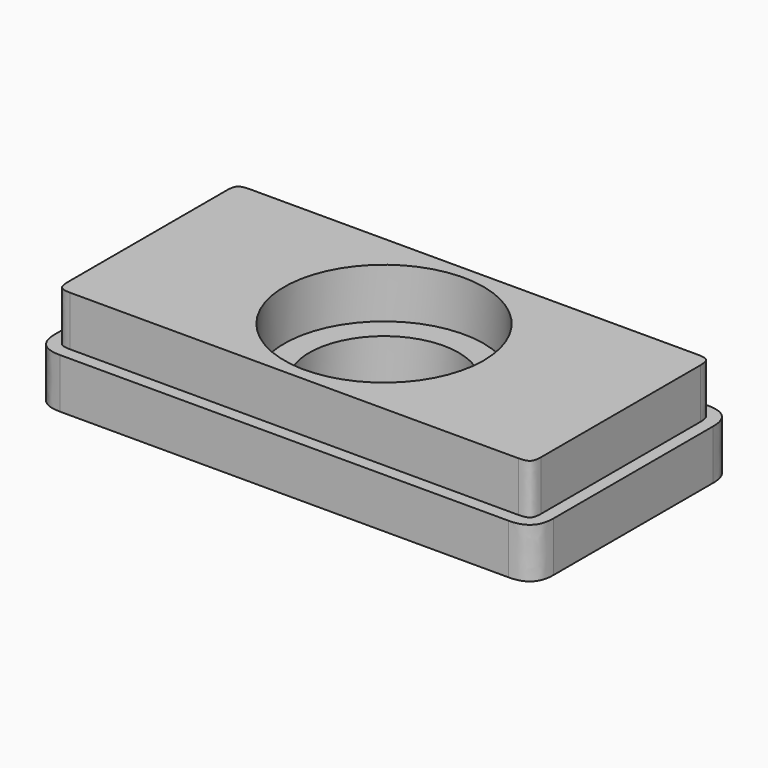
from build123d import *

# Parameters (mm, degrees)
F0_W        = 254
F0_H        = 127
F0_R        = 38.1
F1_DEPTH    = 25.4
F2_T1_DEPTH = 88.9
F3_R        = 50.8
F4_DEPTH    = 25.4


# Not quite as in the source:
# - a fillet or chamfer that OpenCascade refuses, or shapes differently, is made with other operations: its cross-section is extruded or revolved along the edge and cut away or added


with BuildPart() as f1:
    # F0 (on Top) → F1 (new body)
    with BuildSketch(Plane.XY):
        Rectangle(F0_W, F0_H)
        Circle(F0_R, mode=Mode.SUBTRACT)
    extrude(amount=F1_DEPTH)

    # F2: fillet of radius 12.7 on 4 edges, made by hand

    # F2_s2 → F2_t1 (cut)
    with BuildSketch(Plane.XY.offset(-31.75)):
        with BuildLine():
            add(Edge.make_bspline(
                [(114.3, -63.5), (127, -63.5), (127, -50.8)],
                knots=[0, 0, 0, 1, 1, 1], degree=2, weights=[1, 1, 1]))
            Line((127, -50.8), (127, -63.5))
            Line((127, -63.5), (114.3, -63.5))
        make_face()
        with BuildLine():
            add(Edge.make_bspline(
                [(127, 50.8), (127, 63.5), (114.3, 63.5)],
                knots=[0, 0, 0, 1, 1, 1], degree=2, weights=[1, 1, 1]))
            Line((114.3, 63.5), (127, 63.5))
            Line((127, 63.5), (127, 50.8))
        make_face()
        with BuildLine():
            add(Edge.make_bspline(
                [(-127, -50.8), (-127, -63.5), (-114.3, -63.5)],
                knots=[0, 0, 0, 1, 1, 1], degree=2, weights=[1, 1, 1]))
            Line((-114.3, -63.5), (-127, -63.5))
            Line((-127, -63.5), (-127, -50.8))
        make_face()
        with BuildLine():
            add(Edge.make_bspline(
                [(-127, 50.8), (-127, 63.5), (-114.3, 63.5)],
                knots=[0, 0, 0, 1, 1, 1], degree=2, weights=[1, 1, 1]))
            Line((-114.3, 63.5), (-127, 63.5))
            Line((-127, 63.5), (-127, 50.8))
        make_face()
    extrude(amount=F2_T1_DEPTH, mode=Mode.SUBTRACT)

    # F3 (on face) → F4 (join)
    with BuildSketch(Plane.XY.offset(25.4)):
        with BuildLine():
            Line((114.3, 57.1500000767), (-114.3, 57.1500000767))
            add(Edge.make_bspline(
                [(-114.3, 57.1500000767), (-115.0937500032, 57.1500000767), (-116.4821057247, 57.049499097), (-117.9432263511, 56.6940527927), (-118.8342111311, 56.2669565132), (-119.3520160795, 55.8520160795), (-119.7669565132, 55.3342111311), (-120.1940527927, 54.4432263511), (-120.549499097, 52.9821057247), (-120.6500000767, 51.5937500032), (-120.6500000767, 50.8)],
                knots=[0, 0, 0, 0, 0.125, 0.25, 0.375, 0.5, 0.625, 0.75, 0.875, 1, 1, 1, 1], degree=3))
            Line((-120.6500000767, 50.8), (-120.6500000767, -50.8))
            add(Edge.make_bspline(
                [(-120.6500000767, -50.8), (-120.6500000767, -51.5937500032), (-120.549499097, -52.9821057247), (-120.1940527927, -54.4432263511), (-119.7669565132, -55.3342111311), (-119.3520160795, -55.8520160795), (-118.8342111311, -56.2669565132), (-117.9432263511, -56.6940527927), (-116.4821057247, -57.049499097), (-115.0937500032, -57.1500000767), (-114.3, -57.1500000767)],
                knots=[0, 0, 0, 0, 0.125, 0.25, 0.375, 0.5, 0.625, 0.75, 0.875, 1, 1, 1, 1], degree=3))
            Line((-114.3, -57.1500000767), (114.3, -57.1500000767))
            add(Edge.make_bspline(
                [(114.3, -57.1500000767), (115.0937500032, -57.1500000767), (116.4821057247, -57.049499097), (117.9432263511, -56.6940527927), (118.8342111311, -56.2669565132), (119.3520160795, -55.8520160795), (119.7669565132, -55.3342111311), (120.1940527927, -54.4432263511), (120.549499097, -52.9821057247), (120.6500000767, -51.5937500032), (120.6500000767, -50.8)],
                knots=[0, 0, 0, 0, 0.125, 0.25, 0.375, 0.5, 0.625, 0.75, 0.875, 1, 1, 1, 1], degree=3))
            Line((120.6500000767, -50.8), (120.6500000767, 50.8))
            add(Edge.make_bspline(
                [(120.6500000767, 50.8), (120.6500000767, 51.5937500032), (120.549499097, 52.9821057247), (120.1940527927, 54.4432263511), (119.7669565132, 55.3342111311), (119.3520160795, 55.8520160795), (118.8342111311, 56.2669565132), (117.9432263511, 56.6940527927), (116.4821057247, 57.049499097), (115.0937500032, 57.1500000767), (114.3, 57.1500000767)],
                knots=[0, 0, 0, 0, 0.125, 0.25, 0.375, 0.5, 0.625, 0.75, 0.875, 1, 1, 1, 1], degree=3))
        make_face()
        Circle(F3_R, mode=Mode.SUBTRACT)
    extrude(amount=F4_DEPTH)


solid = f1.part
